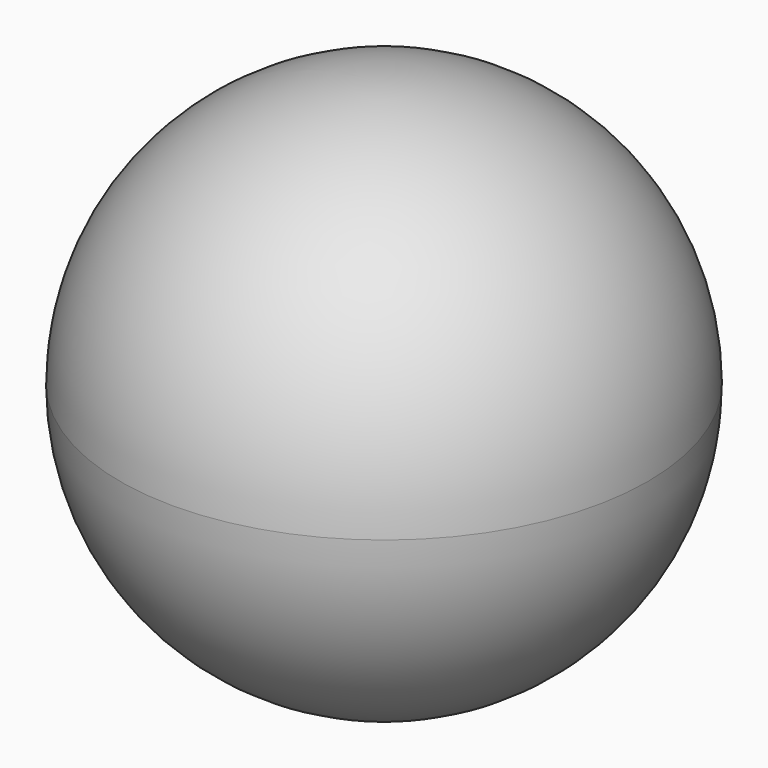
from build123d import *


# Not quite as in the source:
# - the program builds the solid bodies; features that only make, move or delete a surface that nothing else refers to are left out


with BuildPart() as f1:
    # F0 (on Front) → F1 (revolve)
    with BuildSketch(Plane.XZ):
        with BuildLine():
            Line((0, -43.5961931944), (0, 43.5961931944))
            ThreePointArc((0, 43.5961931944), (-30.8271638417, 30.8271638417), (-43.5961931944, 0))
            ThreePointArc((-43.5961931944, 0), (-30.8271638417, -30.8271638417), (0, -43.5961931944))
        make_face()
    revolve(axis=Axis((0, 0, 0), (0, 0, -1)))


solid = f1.part
